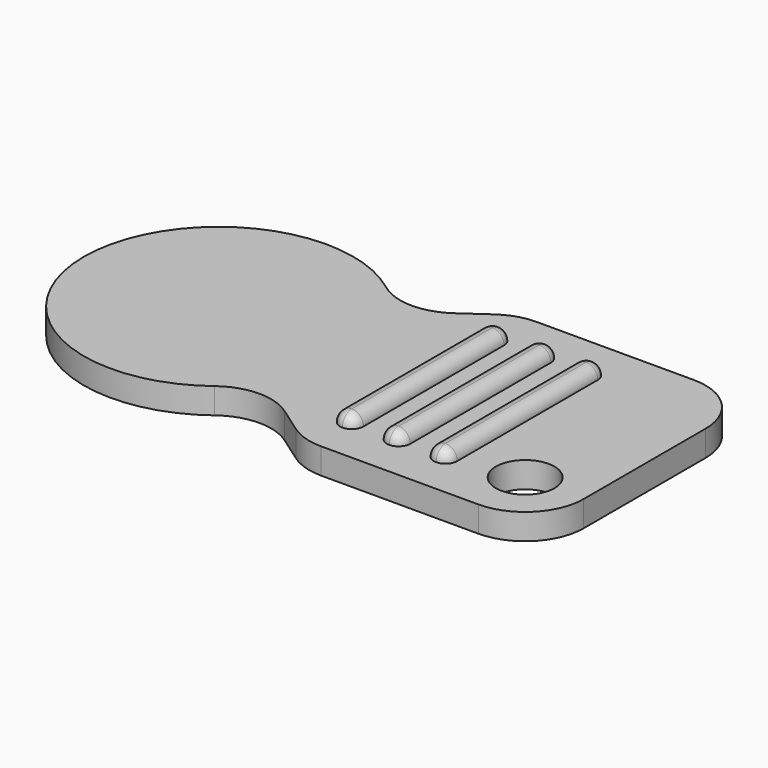
from build123d import *

# Parameters (mm, degrees)
F0_R     = 11.5
F1_DEPTH = 2.2
F3_DEPTH = 2.2
F4_R     = 2.5
F5_DEPTH = 2.201
F6_R     = 5
F7_W     = 2
F7_H     = 17
F8_DEPTH = 1
F9_R     = 0.99999


# Not quite as in the source:
# - a fillet or chamfer is up to 0.001 mm smaller than in the source, because OpenCascade refuses the exact size


with BuildPart() as f1:
    # F0 (on Top) → F1 (new body)
    with BuildSketch(Plane.XY):
        Circle(F0_R)
    extrude(amount=F1_DEPTH)

    # F2 (on Top) → F3 (join)
    with BuildSketch(Plane.XY):
        Polygon((16.363068172, 11.5), (0, 0), (16.363068172, -11.5), (36.363068172, -11.5), (36.363068172, 11.5), align=None)
    extrude(amount=F3_DEPTH)

    # F4 (on face) → F5 (cut, through all)
    with BuildSketch(Plane(origin=(0, 0, 0), x_dir=(1, 0, 0), z_dir=(0, 0, -1))):
        with Locations((31.363068172, 6.5)):
            Circle(F4_R)
    extrude(amount=-F5_DEPTH, mode=Mode.SUBTRACT)

    # F6
    f6_edges = [f1.edges().sort_by_distance(p)[0] for p in [
        (36.363068, -11.5, 1.1),
        (36.363068, 11.5, 1.1),
        (16.363068, -11.5, 1.1),
        (9.408764, -6.6125, 1.1),
        (9.408764, 6.6125, 1.1),
        (16.363068, 11.5, 1.1),
    ]]
    fillet(f6_edges, radius=F6_R)

    # F7 (on face) → F8 (join)
    with BuildSketch(Plane.XY.offset(2.2)):
        with Locations((17.363068172, 0)):
            Rectangle(F7_W, F7_H)
        with Locations((21.363068172, 0)):
            Rectangle(F7_W, F7_H)
        with Locations((25.363068172, 0)):
            Rectangle(F7_W, F7_H)
    extrude(amount=F8_DEPTH)

    # F9 (radius 1 in the source; OpenCascade refuses exactly that, so slightly less here)
    f9_edges = [f1.edges().sort_by_distance(p)[0] for p in [
        (16.363068, -8.5, 2.7),
        (18.363068, -8.5, 2.7),
        (20.363068, -8.5, 2.7),
        (22.363068, -8.5, 2.7),
        (24.363068, -8.5, 2.7),
        (26.363068, -8.5, 2.7),
        (26.363068, 8.5, 2.7),
        (16.363068, 8.5, 2.7),
        (24.363068, 8.5, 2.7),
        (22.363068, 8.5, 2.7),
        (18.363068, 8.5, 2.7),
        (20.363068, 8.5, 2.7),
        (20.363068, 0, 3.2),
        (22.363068, 0, 3.2),
        (21.363068, 8.5, 3.2),
        (21.363068, -8.5, 3.2),
        (18.363068, 0, 3.2),
        (16.363068, 0, 3.2),
        (17.363068, 8.5, 3.2),
        (17.363068, -8.5, 3.2),
        (26.363068, 0, 3.2),
        (24.363068, 0, 3.2),
        (25.363068, 8.5, 3.2),
        (25.363068, -8.5, 3.2),
    ]]
    fillet(f9_edges, radius=F9_R)


solid = f1.part
